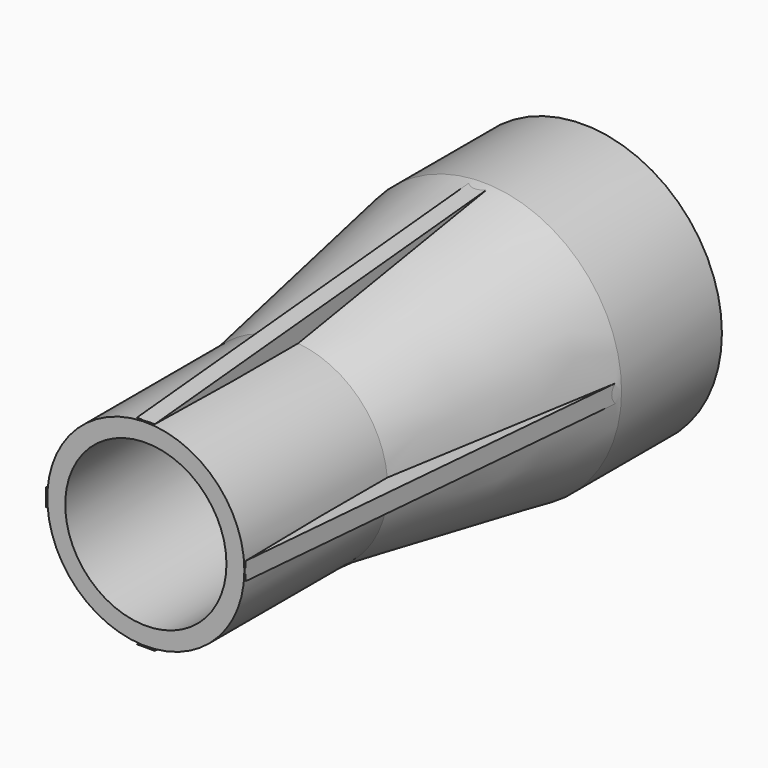
from build123d import *

# Parameters (mm, degrees)
F0_R     = 19.685
F0_R_2   = 17.145
F1_DEPTH = 17.78
F2_W     = 2.54
F2_H     = 25.4
F5_DEPTH = 1.27
F7_COUNT = 2
F7_ANGLE = 90


with BuildPart() as f1:
    # F0 (on Front) → F1 (new body)
    with BuildSketch(Plane.XZ):
        Circle(F0_R)
        Circle(F0_R_2, mode=Mode.SUBTRACT)
    extrude(amount=F1_DEPTH)

    # F2 (on Top) → F3 (revolve)
    with BuildSketch(Plane.XY):
        Polygon((19.685, -17.78), (17.145, -17.78), (11.43, -52.07), (13.97, -52.07), align=None)
        with Locations((12.7, -64.77)):
            Rectangle(F2_W, F2_H)
    revolve(axis=Axis((0, 0, 0), (0, 1, 0)))

    # F4 (on Right) → F5 (join, symmetric)
    with BuildSketch(Plane.YZ):
        Polygon((-17.78, 19.5759806411), (-77.47, 14.1412131567), (-52.3864563458, 13.7231544031), align=None)
        Polygon((-52.3864563458, -13.7231544031), (-77.47, -14.1412131567), (-17.78, -19.5759806411), align=None)
    extrude(amount=F5_DEPTH, both=True)

    # F7: F1 ×2 about axis
    f7_axis = Axis((0, -43.7352471054, 0), (0, -1, 0))


with BuildPart() as f1_1:
    add(f1.part)
    for i in range(1, F7_COUNT):
        add(f1.part.rotate(f7_axis, i * F7_ANGLE / (F7_COUNT - 1)))


solid = f1_1.part
